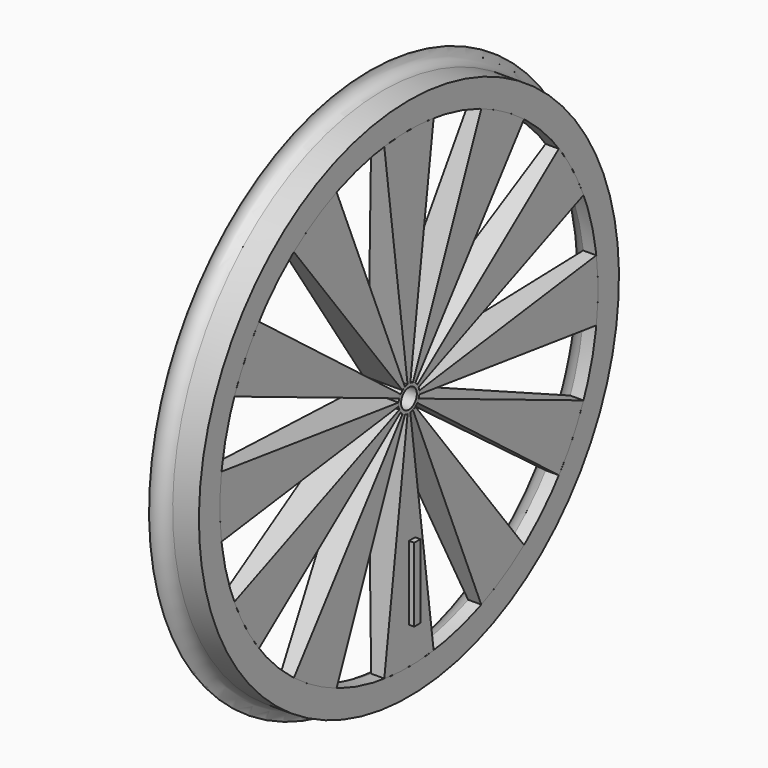
from build123d import *

# Parameters (mm, degrees)
F1_R            = 12.7
F1_R_2          = 9.525
F2_DEPTH        = 38.1
F5_ANGLE_BACK   = 7.5
F5_ANGLE        = 15
F5_COPIES_COUNT = 12
F7_W            = 7.5099463575
F7_H            = 71.462534368
F8_DEPTH        = 5.08


# Not quite as in the source:
# - a pattern or mirror of a feature is missing from the dataset's text; its kind, count and spacing are read off the source's solid


with BuildPart() as f2:
    # F1 (on Right) → F2 (new body)
    with BuildSketch(Plane.YZ):
        Circle(F1_R)
        Circle(F1_R_2, mode=Mode.SUBTRACT)
    extrude(amount=-F2_DEPTH)


with BuildPart() as f3:
    # F0 (on Front) → F3 (revolve)
    with BuildSketch(Plane.XZ):
        with BuildLine():
            Line((0, 228.6), (0, 254))
            Line((0, 254), (-25.4, 254))
            ThreePointArc((-25.4, 254), (-34.3802561211, 257.7197438789), (-38.1, 266.7))
            ThreePointArc((-38.1, 266.7), (-31.7443932738, 243.4204044842), (-12.7, 228.6))
            Line((-12.7, 228.6), (0, 228.6))
        make_face()
    revolve(axis=Axis((-0.2429113246, 0, 0), (1, 0, 0)))


with BuildPart() as f5:
    # F4 (on Front) → F5 (revolve)
    with BuildSketch(Plane.XZ, mode=Mode.PRIVATE) as f5_sk:
        Polygon((0, -228.6), (0, -12.7), (-38.1, -12.7), (-12.7, -228.6), align=None)
    revolve(f5_sk.sketch.rotate(Axis((-28.6667533219, 0, 0), (-1, 0, 0)), -F5_ANGLE_BACK), axis=Axis((-28.6667533219, 0, 0), (-1, 0, 0)), revolution_arc=F5_ANGLE)


with BuildPart() as f5_copies_1:
    # F5_copies: instance of F5
    add(f5.part.rotate(Axis((0, 0, 0), (1, 0, 0)), 1 * 360 / F5_COPIES_COUNT))


with BuildPart() as f5_copies_2:
    # F5_copies: instance of F5
    add(f5.part.rotate(Axis((0, 0, 0), (1, 0, 0)), 2 * 360 / F5_COPIES_COUNT))


with BuildPart() as f5_copies_3:
    # F5_copies: instance of F5
    add(f5.part.rotate(Axis((0, 0, 0), (1, 0, 0)), 3 * 360 / F5_COPIES_COUNT))


with BuildPart() as f5_copies_4:
    # F5_copies: instance of F5
    add(f5.part.rotate(Axis((0, 0, 0), (1, 0, 0)), 4 * 360 / F5_COPIES_COUNT))


with BuildPart() as f5_copies_5:
    # F5_copies: instance of F5
    add(f5.part.rotate(Axis((0, 0, 0), (1, 0, 0)), 5 * 360 / F5_COPIES_COUNT))


with BuildPart() as f5_copies_6:
    # F5_copies: instance of F5
    add(f5.part.rotate(Axis((0, 0, 0), (1, 0, 0)), 6 * 360 / F5_COPIES_COUNT))


with BuildPart() as f5_copies_7:
    # F5_copies: instance of F5
    add(f5.part.rotate(Axis((0, 0, 0), (1, 0, 0)), 7 * 360 / F5_COPIES_COUNT))


with BuildPart() as f5_copies_8:
    # F5_copies: instance of F5
    add(f5.part.rotate(Axis((0, 0, 0), (1, 0, 0)), 8 * 360 / F5_COPIES_COUNT))


with BuildPart() as f5_copies_9:
    # F5_copies: instance of F5
    add(f5.part.rotate(Axis((0, 0, 0), (1, 0, 0)), 9 * 360 / F5_COPIES_COUNT))


with BuildPart() as f5_copies_10:
    # F5_copies: instance of F5
    add(f5.part.rotate(Axis((0, 0, 0), (1, 0, 0)), 10 * 360 / F5_COPIES_COUNT))


with BuildPart() as f5_copies_11:
    # F5_copies: instance of F5
    add(f5.part.rotate(Axis((0, 0, 0), (1, 0, 0)), 11 * 360 / F5_COPIES_COUNT))


with BuildPart() as f5_1:
    add(f5.part)

    # F7 (on Right) → F8 (join)
    with BuildSketch(Plane.YZ):
        with Locations((3.7549731787, -156.9709666073)):
            Rectangle(F7_W, F7_H)
    extrude(amount=F8_DEPTH)


solid = Compound([f2.part, f3.part, f5_copies_1.part, f5_copies_2.part, f5_copies_3.part, f5_copies_4.part, f5_copies_5.part, f5_copies_6.part, f5_copies_7.part, f5_copies_8.part, f5_copies_9.part, f5_copies_10.part, f5_copies_11.part, f5_1.part])
